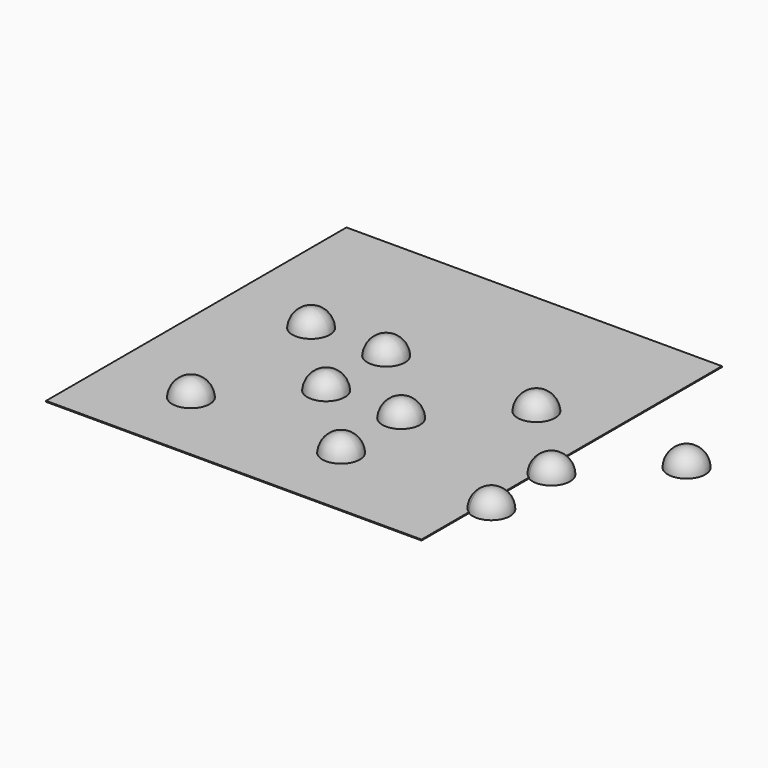
from build123d import *

# Parameters (mm, degrees)
F0_W     = 200
F0_H     = 200
F3_DEPTH = 0.5
F2_R     = 10
F4_DEPTH = 10


# Not quite as in the source:
# - a fillet or chamfer that OpenCascade refuses, or shapes differently, is made with other operations: its cross-section is extruded or revolved along the edge and cut away or added


with BuildPart() as f3:
    # F0 (on Top) → F3 (new body)
    with BuildSketch(Plane.XY):
        Rectangle(F0_W, F0_H)
    extrude(amount=F3_DEPTH)

    # F2 (on face) → F4 (join)
    with BuildSketch(Plane.XY):
        with Locations((-55, -59.7887149453)):
            Circle(F2_R)
        with Locations((-55, 20.2112850547)):
            Circle(F2_R)
        with Locations((-15, -19.7887149453)):
            Circle(F2_R)
        with Locations((-15, 20.2112850547)):
            Circle(F2_R)
        with Locations((25, -59.7887149453)):
            Circle(F2_R)
        with Locations((25, -19.7887149453)):
            Circle(F2_R)
        with Locations((65, 20.2112850547)):
            Circle(F2_R)
        with Locations((105, -59.7887149453)):
            Circle(F2_R)
        with Locations((105, -19.7887149453)):
            Circle(F2_R)
    extrude(amount=F4_DEPTH)

    # F5: fillet of radius 10 on 9 edges, made by hand

    # F5_s1 → F5_t2 (revolve, cut)
    with BuildSketch(Plane.XZ.offset(59.7887149453)):
        with BuildLine():
            ThreePointArc((-45, 0.5), (-48.0954678017, 7.2456883731), (-54.9874921777, 10))
            Line((-54.9874921777, 10), (-45, 10))
            Line((-45, 10), (-45, 0.5))
        make_face()
    revolve(axis=Axis((-55, -59.7887149453, 10), (0, 0, 1)), mode=Mode.SUBTRACT)

    # F5_s3 → F5_t4 (revolve, cut)
    with BuildSketch(Plane.XZ.offset(19.7887149453)):
        with BuildLine():
            ThreePointArc((-5, 0.5), (-8.0954678017, 7.2456883731), (-14.9874921777, 10))
            Line((-14.9874921777, 10), (-5, 10))
            Line((-5, 10), (-5, 0.5))
        make_face()
    revolve(axis=Axis((-15, -19.7887149453, 10), (0, 0, 1)), mode=Mode.SUBTRACT)

    # F5_s5 → F5_t6 (revolve, cut)
    with BuildSketch(Plane.XZ.offset(-20.2112850547)):
        with BuildLine():
            ThreePointArc((-5, 0.5), (-8.0954678017, 7.2456883731), (-14.9874921777, 10))
            Line((-14.9874921777, 10), (-5, 10))
            Line((-5, 10), (-5, 0.5))
        make_face()
    revolve(axis=Axis((-15, 20.2112850547, 10), (0, 0, 1)), mode=Mode.SUBTRACT)

    # F5_s7 → F5_t8 (revolve, cut)
    with BuildSketch(Plane.XZ.offset(-20.2112850547)):
        with BuildLine():
            ThreePointArc((-45, 0.5), (-48.0954678017, 7.2456883731), (-54.9874921777, 10))
            Line((-54.9874921777, 10), (-45, 10))
            Line((-45, 10), (-45, 0.5))
        make_face()
    revolve(axis=Axis((-55, 20.2112850547, 10), (0, 0, 1)), mode=Mode.SUBTRACT)

    # F5_s9 → F5_t10 (revolve, cut)
    with BuildSketch(Plane.XZ.offset(-20.2112850547)):
        with BuildLine():
            ThreePointArc((75, 0.5), (71.9045321983, 7.2456883731), (65.0125078223, 10))
            Line((65.0125078223, 10), (75, 10))
            Line((75, 10), (75, 0.5))
        make_face()
    revolve(axis=Axis((65, 20.2112850547, 10), (0, 0, 1)), mode=Mode.SUBTRACT)

    # F5_s11 → F5_t12 (revolve, cut)
    with BuildSketch(Plane.XZ.offset(19.7887149453)):
        with BuildLine():
            ThreePointArc((35, 0.5), (31.9045321983, 7.2456883731), (25.0125078223, 10))
            Line((25.0125078223, 10), (35, 10))
            Line((35, 10), (35, 0.5))
        make_face()
    revolve(axis=Axis((25, -19.7887149453, 10), (0, 0, 1)), mode=Mode.SUBTRACT)

    # F5_s13 → F5_t14 (revolve, cut)
    with BuildSketch(Plane.XZ.offset(59.7887149453)):
        with BuildLine():
            ThreePointArc((35, 0.5), (31.9045321983, 7.2456883731), (25.0125078223, 10))
            Line((25.0125078223, 10), (35, 10))
            Line((35, 10), (35, 0.5))
        make_face()
    revolve(axis=Axis((25, -59.7887149453, 10), (0, 0, 1)), mode=Mode.SUBTRACT)


with BuildPart() as f4:
    # F2 (on face) → F4, piece 2 (new body)
    with BuildSketch(Plane.XY):
        with Locations((145, 20.2112850547)):
            Circle(F2_R)
    extrude(amount=F4_DEPTH)

    # F5#2: fillet of radius 10 on 1 edges, made by hand

    # F5_2_s1 → F5_2_t2 (revolve, cut)
    with BuildSketch(Plane.XZ.offset(-20.2112850547)):
        with BuildLine():
            ThreePointArc((155, 0), (152.0710678119, 7.0710678119), (145, 10))
            Line((145, 10), (155, 10))
            Line((155, 10), (155, 0))
        make_face()
    revolve(axis=Axis((145, 20.2112850547, 10), (0, 0, 1)), mode=Mode.SUBTRACT)


with BuildPart() as f5_tool16:
    # F5_s17 → F5_t18 (revolve)
    with BuildSketch(Plane.XZ.offset(19.7887149453)):
        with BuildLine():
            ThreePointArc((115, 0), (112.0710678119, 7.0710678119), (105, 10))
            Line((105, 10), (115, 10))
            Line((115, 10), (115, 0))
        make_face()
    revolve(axis=Axis((105, -19.7887149453, 10), (0, 0, 1)))

    split(bisect_by=Plane.YZ.offset(100), keep=Keep.TOP)


with BuildPart() as f3_1:
    add(f3.part)

    # F5_t15: cut F5_tool16
    add(f5_tool16.part, mode=Mode.SUBTRACT)


with BuildPart() as f5_tool21:
    # F5_s22 → F5_t23 (revolve)
    with BuildSketch(Plane.XZ.offset(19.7887149453)):
        with BuildLine():
            ThreePointArc((115, 0), (112.0710678119, 7.0710678119), (105, 10))
            Line((105, 10), (115, 10))
            Line((115, 10), (115, 0))
        make_face()
    revolve(axis=Axis((105, -19.7887149453, 10), (0, 0, 1)))

    split(bisect_by=Plane.XY.offset(0.5), keep=Keep.TOP)


with BuildPart() as f3_2:
    add(f3_1.part)

    # F5_t20: cut F5_tool21
    add(f5_tool21.part, mode=Mode.SUBTRACT)


with BuildPart() as f5_tool26:
    # F5_s27 → F5_t28 (revolve)
    with BuildSketch(Plane.XZ.offset(59.7887149453)):
        with BuildLine():
            ThreePointArc((115, 0), (112.0710678119, 7.0710678119), (105, 10))
            Line((105, 10), (115, 10))
            Line((115, 10), (115, 0))
        make_face()
    revolve(axis=Axis((105, -59.7887149453, 10), (0, 0, 1)))

    split(bisect_by=Plane.YZ.offset(100), keep=Keep.TOP)


with BuildPart() as f3_3:
    add(f3_2.part)

    # F5_t25: cut F5_tool26
    add(f5_tool26.part, mode=Mode.SUBTRACT)


with BuildPart() as f5_tool31:
    # F5_s32 → F5_t33 (revolve)
    with BuildSketch(Plane.XZ.offset(59.7887149453)):
        with BuildLine():
            ThreePointArc((115, 0), (112.0710678119, 7.0710678119), (105, 10))
            Line((105, 10), (115, 10))
            Line((115, 10), (115, 0))
        make_face()
    revolve(axis=Axis((105, -59.7887149453, 10), (0, 0, 1)))

    split(bisect_by=Plane.XY.offset(0.5), keep=Keep.TOP)


with BuildPart() as f3_4:
    add(f3_3.part)

    # F5_t30: cut F5_tool31
    add(f5_tool31.part, mode=Mode.SUBTRACT)


solid = Compound([f4.part, f3_4.part])
